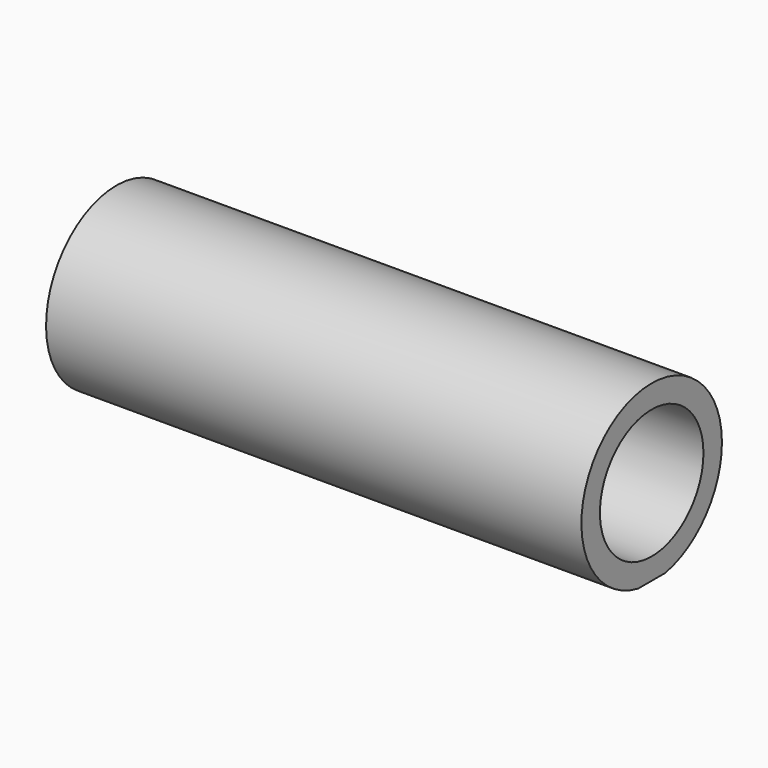
from build123d import *

# Parameters (mm, degrees)
F0_R     = 9.169002
F1_DEPTH = 76.2


# Not quite as in the source:
# - a fillet or chamfer that OpenCascade refuses, or shapes differently, is made with other operations: its cross-section is extruded or revolved along the edge and cut away or added


with BuildPart() as f1:
    # F0 (on Right) → F1 (new body)
    with BuildSketch(Plane.YZ):
        with BuildLine():
            ThreePointArc((2.414251, -12.206699), (9.61439, -7.899089), (12.443155, 0))
            ThreePointArc((12.443155, 0), (-7.899089, 9.61439), (-2.414251, -12.206699))
            Line((-2.414251, -12.206699), (0, -12.206699))
            Line((0, -12.206699), (2.414251, -12.206699))
        make_face()
        Circle(F0_R, mode=Mode.SUBTRACT)
    extrude(amount=F1_DEPTH)

    # F2: fillet of radius 5.08 on 1 edges, made by hand

    # F2_s1 → F2_t2 (revolve, cut)
    with BuildSketch(Plane.XY):
        with BuildLine():
            ThreePointArc((0, 14.249002), (1.487898, 10.6569), (5.08, 9.169002))
            Line((5.08, 9.169002), (0, 9.169002))
            Line((0, 9.169002), (0, 14.249002))
        make_face()
    revolve(axis=Axis((0, 0, 0), (1, 0, 0)), mode=Mode.SUBTRACT)


solid = f1.part
